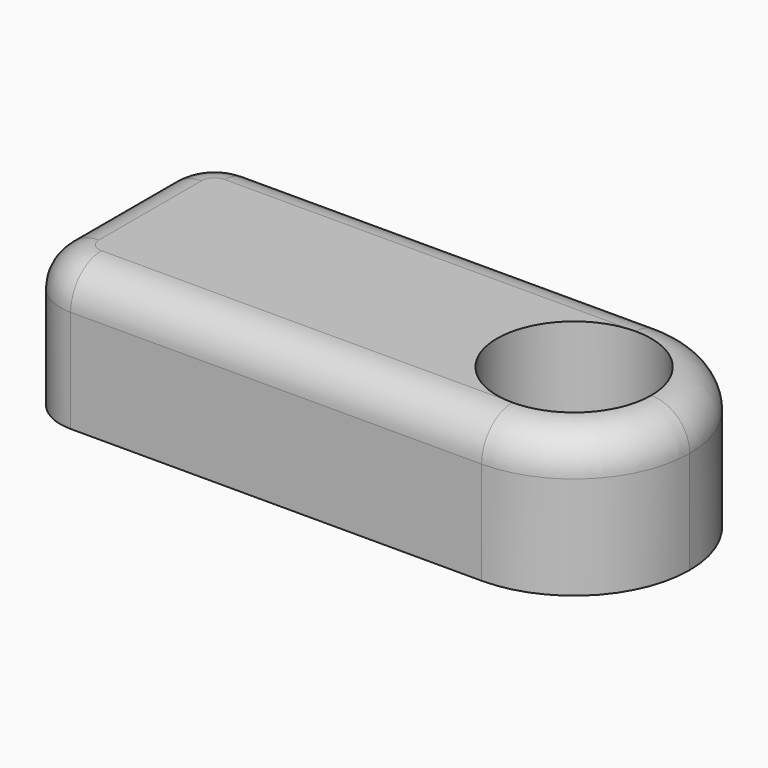
from build123d import *

# Parameters (mm, degrees)
F0_W     = 22.5
F0_H     = 9
F1_DEPTH = 5.5
F2_R     = 3
F3_DEPTH = 3.25
F4_R     = 1.6
F5_DEPTH = 2.5
F6_R     = 4.49999
F7_R     = 2
F8_R     = 1.49999


# Not quite as in the source:
# - a fillet or chamfer is up to 0.001 mm smaller than in the source, because OpenCascade refuses the exact size


with BuildPart() as f1:
    # F0 (on Top) → F1 (new body)
    with BuildSketch(Plane.XY):
        with Locations((-6.75, 0)):
            Rectangle(F0_W, F0_H)
    extrude(amount=F1_DEPTH)

    # F2 (on face) → F3 (cut)
    with BuildSketch(Plane.XY.offset(5.5)):
        Circle(F2_R)
    extrude(amount=-F3_DEPTH, mode=Mode.SUBTRACT)

    # F4 (on face) → F5 (cut)
    with BuildSketch(Plane.XY.offset(2.25)):
        Circle(F4_R)
    extrude(amount=-F5_DEPTH, mode=Mode.SUBTRACT)

    # F6 (radius 4.5 in the source; OpenCascade refuses exactly that, so slightly less here)
    f6_edges = [f1.edges().sort_by_distance(p)[0] for p in [
        (4.5, -4.5, 2.75),
        (4.5, 4.5, 2.75),
    ]]
    fillet(f6_edges, radius=F6_R)

    # F7
    f7_edges = [f1.edges().sort_by_distance(p)[0] for p in [
        (-18, 4.5, 2.75),
        (-18, -4.5, 2.75),
    ]]
    fillet(f7_edges, radius=F7_R)

    # F8 (radius 1.5 in the source; OpenCascade refuses exactly that, so slightly less here)
    f8_edges = [f1.edges().sort_by_distance(p)[0] for p in [
        (-7.999995, -4.5, 5.5),
    ]]
    fillet(f8_edges, radius=F8_R)


solid = f1.part
